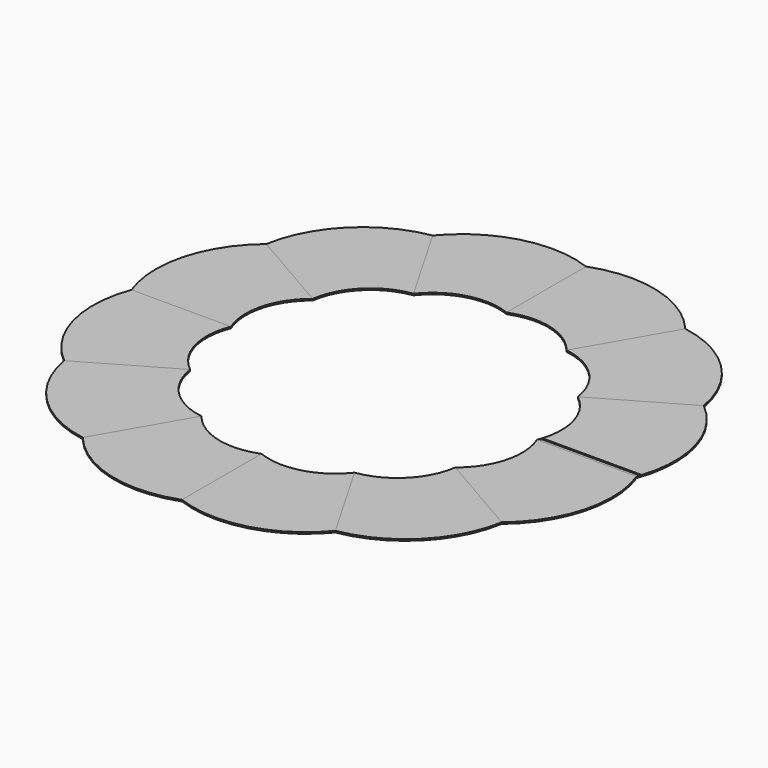
from build123d import *

# Parameters (mm, degrees)
F1_DEPTH               = 5
F3_COUNT               = 12
F5_DEPTH               = 2
DRAFT_F5_DRAFTED_ANGLE = 45


# Not quite as in the source:
# - an extrude with a draft is written as a straight extrude whose walls are then drafted


with BuildPart() as f1:
    # F0 (on Top) → F1 (new body)
    with BuildSketch(Plane.XY):
        with BuildLine():
            Line((523.1785178185, 0), (825, 0))
            ThreePointArc((825, 0), (835.4751134397, 223.8648819425), (714.4709581222, 412.5))
            Line((714.4709581222, 412.5), (433.0127018922, 250))
            ThreePointArc((433.0127018922, 250), (508.0781786008, 136.139137648), (500, 0))
            Line((500, 0), (523.1785178185, 0))
        make_face()
    extrude(amount=F1_DEPTH)


with BuildPart() as f3_1:
    # F3: instance of F1
    add(f1.part.rotate(Axis((0, 0, -9.5117650926), (0, 0, -1)), 1 * 360 / F3_COUNT))


with BuildPart() as f3_2:
    # F3: instance of F1
    add(f1.part.rotate(Axis((0, 0, -9.5117650926), (0, 0, -1)), 2 * 360 / F3_COUNT))


with BuildPart() as f3_3:
    # F3: instance of F1
    add(f1.part.rotate(Axis((0, 0, -9.5117650926), (0, 0, -1)), 3 * 360 / F3_COUNT))


with BuildPart() as f3_4:
    # F3: instance of F1
    add(f1.part.rotate(Axis((0, 0, -9.5117650926), (0, 0, -1)), 4 * 360 / F3_COUNT))


with BuildPart() as f3_5:
    # F3: instance of F1
    add(f1.part.rotate(Axis((0, 0, -9.5117650926), (0, 0, -1)), 5 * 360 / F3_COUNT))


with BuildPart() as f3_6:
    # F3: instance of F1
    add(f1.part.rotate(Axis((0, 0, -9.5117650926), (0, 0, -1)), 6 * 360 / F3_COUNT))


with BuildPart() as f3_7:
    # F3: instance of F1
    add(f1.part.rotate(Axis((0, 0, -9.5117650926), (0, 0, -1)), 7 * 360 / F3_COUNT))


with BuildPart() as f3_8:
    # F3: instance of F1
    add(f1.part.rotate(Axis((0, 0, -9.5117650926), (0, 0, -1)), 8 * 360 / F3_COUNT))


with BuildPart() as f3_9:
    # F3: instance of F1
    add(f1.part.rotate(Axis((0, 0, -9.5117650926), (0, 0, -1)), 9 * 360 / F3_COUNT))


with BuildPart() as f3_10:
    # F3: instance of F1
    add(f1.part.rotate(Axis((0, 0, -9.5117650926), (0, 0, -1)), 10 * 360 / F3_COUNT))


with BuildPart() as f3_11:
    # F3: instance of F1
    add(f1.part.rotate(Axis((0, 0, -9.5117650926), (0, 0, -1)), 11 * 360 / F3_COUNT))


with BuildPart() as f5_drafted:
    # F4 (on face) → F5 (new body)
    with BuildSketch(Plane.XY.offset(5)):
        with BuildLine():
            ThreePointArc((505.2743949768, 14.7157625851), (503.8785536147, 10.4794912124), (502.3955679352, 6.2729342206))
            Line((502.3955679352, 6.2729342206), (827.2633811999, 6.2729342206))
            ThreePointArc((827.2633811999, 6.2729342206), (828.7120523706, 10.4857568074), (830.1097552825, 14.7157625851))
            Line((830.1097552825, 14.7157625851), (505.2743949768, 14.7157625851))
        make_face()
    extrude(amount=-F5_DEPTH)

    # draft_F5_drafted
    draft_f5_drafted_walls = [f5_drafted.faces().sort_by_distance(p)[0] for p in [
        (828.7120523706, 10.4857568074, 3.6666666667),
        (667.6920751296, 14.7157625851, 3.6666666667),
        (503.8785536147, 10.4794912124, 3.6666666667),
        (664.8294745676, 6.2729342206, 3.6666666667),
    ]]
    draft(draft_f5_drafted_walls, neutral_plane=Plane(origin=(0, 0, 5), x_dir=(1, 0, 0), z_dir=(0, 0, -1)), angle=DRAFT_F5_DRAFTED_ANGLE)


with BuildPart() as f1_1:
    add(f1.part)

    # join_F5_drafted: cut F5_drafted
    add(f5_drafted.part, mode=Mode.SUBTRACT)


solid = Compound([f3_1.part, f3_2.part, f3_3.part, f3_4.part, f3_5.part, f3_6.part, f3_7.part, f3_8.part, f3_9.part, f3_10.part, f3_11.part, f1_1.part])
